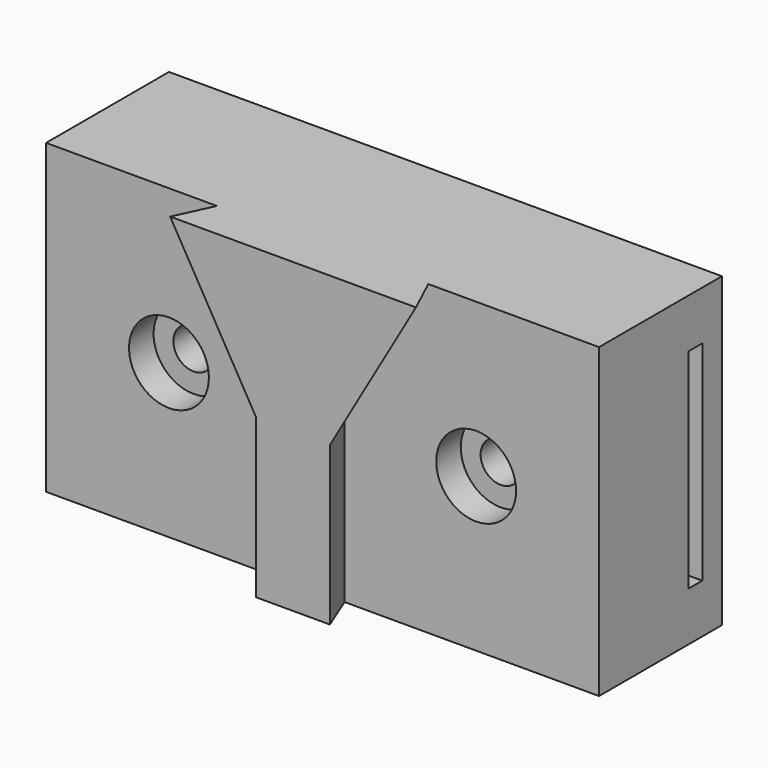
from build123d import *

# Parameters (mm, degrees)
F0_W      = 31.75
F0_H      = 63.5
F1_DEPTH  = 114.3
F2_DEPTH  = 114.3
F4_D      = 8.334375
F4_2_D    = 8.334375
F7_DEPTH  = 7.62
F8_W      = 3.556
F8_H      = 43.18
F9_DEPTH  = 38.1
F10_START = 76.2
F10_DEPTH = 38.1
F14_R     = 8.255
F14_R_2   = 4.1671875
F15_R     = 8.255
F15_R_2   = 4.1671875
F16_DEPTH = 6.35
F17_R     = 4.1671875
F18_DEPTH = 4.2672


# Not quite as in the source:
# - a length typed as a fraction of an inch, garbled in the dataset ("3 / 203.2 mm" for 3/8 in), is restored


with BuildPart() as f1:
    # F0 (on Right) → F1 (new body)
    with BuildSketch(Plane.YZ):
        with Locations((20.6751725854, 0)):
            Rectangle(F0_W, F0_H)
    extrude(amount=F1_DEPTH)

    # F4 (through all)
    with Locations(Plane.XZ.offset(26.9498274146)):
        with Locations((25.4, 0), (88.9, 0)):
            Hole(F4_D / 2)

    # F6 (on face) → F7 (join)
    with BuildSketch(Plane.XZ.offset(-4.8001725854)):
        Polygon((57.15, -31.75), (57.15, 31.75), (31.75, 31.75), (49.53, 0.9541366414), (49.53, -31.75), align=None)
        Polygon((82.55, 31.75), (57.15, 31.75), (57.15, -31.75), (64.77, -31.75), (64.77, 0.9541366414), align=None)
    extrude(amount=F7_DEPTH)

    # F8 (on face) → F9 (cut)
    with BuildSketch(Plane.YZ):
        with Locations((29.6921725854, 0)):
            Rectangle(F8_W, F8_H)
    extrude(amount=F9_DEPTH, mode=Mode.SUBTRACT)

    # F8 (on face) → F10 (cut)
    with BuildSketch(Plane.YZ.offset(F10_START)):
        with Locations((29.6921725854, 0)):
            Rectangle(F8_W, F8_H)
    extrude(amount=F10_DEPTH, mode=Mode.SUBTRACT)

    # F12: sweep along a path in F12_path
    with BuildLine(Plane(origin=(31.75, -2.8198274146, 31.75), x_dir=(0, 0, 1), z_dir=(0, -1, 0))) as f12_path:
        Line((0, 0), (-30.7958633586, -17.78))
        Line((-30.7958633586, -17.78), (-63.5, -17.78))
    # F11 (on face) → F12 (sweep, cut)
    with BuildSketch(Plane.XY.offset(31.75)):
        Polygon((35.306, 4.8001725854), (31.75, 4.8001725854), (31.75, -2.8198274146), align=None)
    sweep(path=f12_path.line, transition=Transition.RIGHT, mode=Mode.SUBTRACT)

    # F13: sweep along a path in F13_path
    with BuildLine(Plane(origin=(82.55, -2.8198274146, 31.75), x_dir=(0, 0, -1), z_dir=(0, 1, 0))) as f13_path:
        Line((0, 0), (30.7958633586, 17.78))
        Line((30.7958633586, 17.78), (63.5, 17.78))
    # F11 (on face) → F13 (sweep, cut)
    with BuildSketch(Plane.XY.offset(31.75)):
        Polygon((78.994, 4.8001725854), (82.55, -2.8198274146), (82.55, 4.8001725854), align=None)
    sweep(path=f13_path.line, transition=Transition.RIGHT, mode=Mode.SUBTRACT)

    # F14 (on face) + F15 (on face) → F16 (cut)
    with BuildSketch(Plane.XZ.offset(-4.8001725854)):
        with Locations((25.4, 0)):
            Circle(F14_R)
        with Locations((25.4, 0)):
            Circle(F14_R_2, mode=Mode.SUBTRACT)
    with BuildSketch(Plane.XZ.offset(-4.8001725854)):
        with Locations((88.9, 0)):
            Circle(F15_R)
        with Locations((88.9, 0)):
            Circle(F15_R_2, mode=Mode.SUBTRACT)
    extrude(amount=-F16_DEPTH, mode=Mode.SUBTRACT)

    # F17 (on face) → F18 (cut)
    with BuildSketch(Plane(origin=(0, 36.5501725854, 0), x_dir=(-1, 0, 0), z_dir=(0, 1, 0))):
        Polygon((-83.4644, -3.1382451232), (-83.4644, 3.1382451232), (-88.9, 6.2764902464), (-94.3356, 3.1382451232), (-94.3356, -3.1382451232), (-88.9, -6.2764902464), align=None)
        with Locations((-88.9, 0)):
            Circle(F17_R, mode=Mode.SUBTRACT)
        Polygon((-30.8356, 3.1382451232), (-30.8356, -3.1382451232), (-25.4, -6.2764902464), (-19.9644, -3.1382451232), (-19.9644, 3.1382451232), (-25.4, 6.2764902464), align=None)
        with Locations((-25.4, 0)):
            Circle(F17_R, mode=Mode.SUBTRACT)
    extrude(amount=-F18_DEPTH, mode=Mode.SUBTRACT)


with BuildPart() as f2:
    # F0 (on Right) → F2 (new body)
    with BuildSketch(Plane.YZ):
        Polygon((-26.9498274146, -19.685), (-26.9498274146, -31.75), (4.8001725854, -31.75), (4.8001725854, 31.75), (-26.9498274146, 31.75), (-26.9498274146, 19.685), (-23.3938274146, 19.685), (-7.8998274146, 8.89), (-7.8998274146, -8.89), (-23.3938274146, -19.685), align=None)
        Polygon((-26.9498274146, 19.685), (-26.9498274146, -19.685), (-23.3938274146, -19.685), (-7.8998274146, -8.89), (-7.8998274146, 8.89), (-23.3938274146, 19.685), align=None)
    extrude(amount=F2_DEPTH)

    # F4#2 (through all)
    with Locations(Plane.XZ.offset(26.9498274146)):
        with Locations((25.4, 0), (88.9, 0)):
            Hole(F4_2_D / 2)


solid = f1.part
